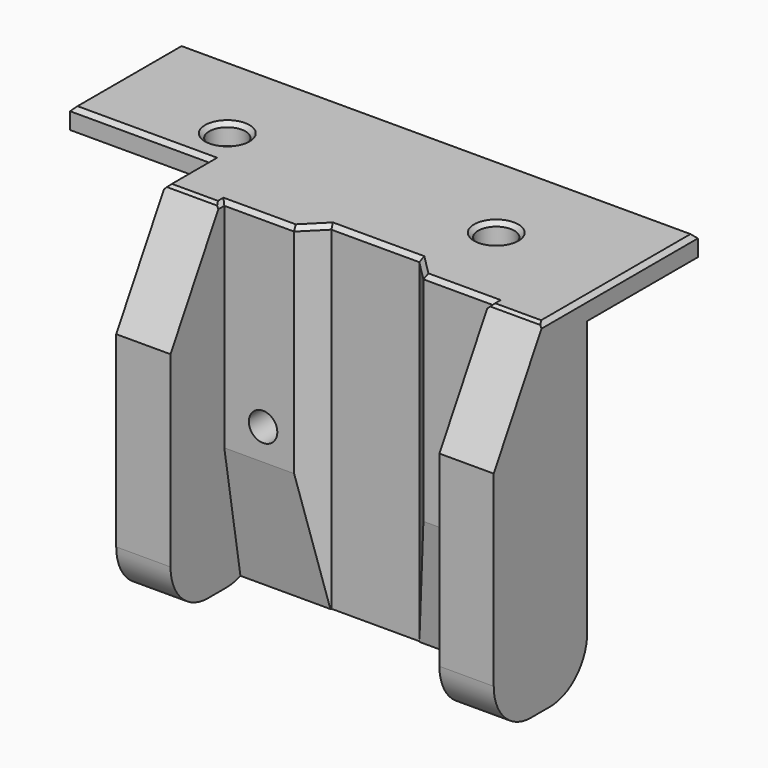
from build123d import *

# Parameters (mm, degrees)
F0_W           = 13.375
F0_H           = 2
F1_DEPTH       = 25
F2_R           = 1.75
F3_DEPTH       = 2
F4_W           = 11.3
F4_H           = 33
F5_DEPTH       = 25
F5_DEPTH_BACK  = 11.5
F6_W           = 26
F6_H           = 6.5
F7_DEPTH       = 33
F9_DEPTH       = 33
F11_DEPTH      = 19.75
F11_DEPTH_BACK = 6.25
F12_R          = 1.375
F13_DEPTH      = 4.8
F14_W          = 5.5
F14_H          = 5.5
F15_DEPTH      = 1.5
F16_T1_DEPTH   = 27.75
F16_T3_DEPTH   = 27.75
F16_T5_DEPTH   = 59
F17_T1_DEPTH   = 59.021567647
F17_T3_DEPTH   = 59.021567647
F18_T1_DEPTH   = 6.4746360003
F18_T3_DEPTH   = 20.7323463904
F18_T5_DEPTH   = 52.0573463904
F18_T7_DEPTH   = 15.4323463904
F18_T9_DEPTH   = 14.5286731952
F18_T11_DEPTH  = 6.3286731952
F18_T13_DEPTH  = 6.4746360003
F18_T15_DEPTH  = 1.5286731952
F18_T17_DEPTH  = 7.7786731952
F18_T19_DEPTH  = 7.7786731952
F18_T24_DEPTH  = 4.8857735151
F18_T29_DEPTH  = 10.5573463904
F18_T35_DEPTH  = 4.8857735151
F18_T45_DEPTH  = 14.5286731952
F18_T49_DEPTH  = 7.3573463904
F18_T56_DEPTH  = 8.8073463904
F18_T60_DEPTH  = 2.5573463904
F18_T67_DEPTH  = 4.8857735151
F18_T71_DEPTH  = 10.5573463904
F18_T78_DEPTH  = 10.5573463904
F18_T82_DEPTH  = 4.8857735151
F18_T89_DEPTH  = 2.5573463904
F18_T93_DEPTH  = 8.8073463904


# Not quite as in the source:
# - a fillet or chamfer that OpenCascade refuses, or shapes differently, is made with other operations: its cross-section is extruded or revolved along the edge and cut away or added


with BuildPart() as f1:
    # F0 (on Right) → F1 (new body, symmetric)
    with BuildSketch(Plane.YZ):
        with Locations((6.6875, 1)):
            Rectangle(F0_W, F0_H)
    extrude(amount=F1_DEPTH, both=True)

    # F2 (on face) → F3 (cut, through all)
    with BuildSketch(Plane.XY.offset(2)):
        with Locations((-13, 4)):
            Circle(F2_R)
        with Locations((13, 4)):
            Circle(F2_R)
    extrude(amount=-F3_DEPTH, mode=Mode.SUBTRACT)

    # F4 (on Right) → F5 (join, two sides)
    with BuildSketch(Plane.YZ) as f5_sk:
        with Locations((-5.65, -14.5)):
            Rectangle(F4_W, F4_H)
    extrude(amount=F5_DEPTH)
    extrude(f5_sk.sketch, amount=-F5_DEPTH_BACK)

    # F6 (on face) → F7 (cut, through all)
    with BuildSketch(Plane(origin=(0, 0, -31), x_dir=(1, 0, 0), z_dir=(0, 0, -1))):
        with Locations((6.75, 8.05)):
            Rectangle(F6_W, F6_H)
    extrude(amount=-F7_DEPTH, mode=Mode.SUBTRACT)

    # F8 (on face) → F9 (cut, through all)
    with BuildSketch(Plane(origin=(0, 0, -31), x_dir=(1, 0, 0), z_dir=(0, 0, -1))):
        Polygon((13, 4.8), (0.5, 4.8), (2.5, 2.8), (11, 2.8), align=None)
    extrude(amount=-F9_DEPTH, mode=Mode.SUBTRACT)

    # F10 (on Right) → F11 (cut, two sides)
    with BuildSketch(Plane.YZ) as f11_sk:
        Polygon((-4.8, -31), (-2.8, -31), (-4.8, -19), align=None)
    extrude(amount=F11_DEPTH, mode=Mode.SUBTRACT)
    extrude(f11_sk.sketch, amount=-F11_DEPTH_BACK, mode=Mode.SUBTRACT)

    # F12 (on face) → F13 (cut, through all)
    with BuildSketch(Plane.XZ.offset(4.8)):
        with Locations((-2.5, -16)):
            Circle(F12_R)
        with Locations((16, -16)):
            Circle(F12_R)
    extrude(amount=-F13_DEPTH, mode=Mode.SUBTRACT)

    # F14 (on face) → F15 (cut)
    with BuildSketch(Plane(origin=(0, 0, 0), x_dir=(-1, 0, 0), z_dir=(0, 1, 0))):
        with Locations((-16, -16)):
            Rectangle(F14_W, F14_H)
        with Locations((2.5, -16)):
            Rectangle(F14_W, F14_H)
    extrude(amount=-F15_DEPTH, mode=Mode.SUBTRACT)

    # F16: fillet of radius 4.5 on 3 edges, made by hand

    # F16_s2 → F16_t1 (cut)
    with BuildSketch(Plane.YZ.offset(-22.75)):
        with BuildLine():
            ThreePointArc((-11.3, -26.5), (-9.9819805153, -29.6819805153), (-6.8, -31))
            Line((-6.8, -31), (-11.3, -31))
            Line((-11.3, -31), (-11.3, -26.5))
        make_face()
    extrude(amount=F16_T1_DEPTH, mode=Mode.SUBTRACT)

    # F16_s4 → F16_t3 (cut)
    with BuildSketch(Plane.YZ.offset(8.5)):
        with BuildLine():
            ThreePointArc((-11.3, -26.5), (-9.9819805153, -29.6819805153), (-6.8, -31))
            Line((-6.8, -31), (-11.3, -31))
            Line((-11.3, -31), (-11.3, -26.5))
        make_face()
    extrude(amount=F16_T3_DEPTH, mode=Mode.SUBTRACT)

    # F16_s6 → F16_t5 (cut)
    with BuildSketch(Plane.YZ.offset(-22.75)):
        with BuildLine():
            ThreePointArc((0, -26.5), (-1.3180194847, -29.6819805153), (-4.5, -31))
            Line((-4.5, -31), (0, -31))
            Line((0, -31), (0, -26.5))
        make_face()
    extrude(amount=F16_T5_DEPTH, mode=Mode.SUBTRACT)

    # F17: chamfer of 6 x 10.3923048454 on 2 edges, made by hand

    # F17_s2 → F17_t1 (cut)
    with BuildSketch(Plane.YZ.offset(-38.3857838235)):
        Polygon((-5.3, 2), (-11.3, -8.3923048454), (-11.3, 2), align=None)
    extrude(amount=F17_T1_DEPTH, mode=Mode.SUBTRACT)

    # F17_s4 → F17_t3 (cut)
    with BuildSketch(Plane.YZ.offset(-7.1357838235)):
        Polygon((-5.3, 2), (-11.3, -8.3923048454), (-11.3, 2), align=None)
    extrude(amount=F17_T3_DEPTH, mode=Mode.SUBTRACT)

    # F18: chamfer of 0.4 on 16 edges, made by hand

    # F18_s2 → F18_t1 (cut)
    with BuildSketch(Plane.YZ.offset(19.1376819998)):
        Polygon((-5.4154700538, 1.8), (-5.0690598923, 2), (-5.3, 2), align=None)
    extrude(amount=F18_T1_DEPTH, mode=Mode.SUBTRACT)

    # F18_s4 → F18_t3 (cut)
    with BuildSketch(Plane.XZ.offset(-14.4036731952)):
        Polygon((25, 1.6), (24.6, 2), (25, 2), align=None)
    extrude(amount=F18_T3_DEPTH, mode=Mode.SUBTRACT)

    # F18_s6 → F18_t5 (cut)
    with BuildSketch(Plane.YZ.offset(-26.0286731952)):
        Polygon((13.375, 1.6), (12.975, 2), (13.375, 2), align=None)
    extrude(amount=F18_T5_DEPTH, mode=Mode.SUBTRACT)

    # F18_s8 → F18_t7 (cut)
    with BuildSketch(Plane.XZ.offset(-14.4036731952)):
        Polygon((-25, 1.6), (-24.6, 2), (-25, 2), align=None)
    extrude(amount=F18_T7_DEPTH, mode=Mode.SUBTRACT)

    # F18_s10 → F18_t9 (cut)
    with BuildSketch(Plane.YZ.offset(-26.0286731952)):
        Polygon((0, 1.6), (0.4, 2), (0, 2), align=None)
    extrude(amount=F18_T9_DEPTH, mode=Mode.SUBTRACT)

    # F18_s12 → F18_t11 (cut)
    with BuildSketch(Plane.XZ):
        Polygon((-11.5, 1.6), (-11.1, 2), (-11.5, 2), align=None)
    extrude(amount=F18_T11_DEPTH, mode=Mode.SUBTRACT)

    # F18_s14 → F18_t13 (cut)
    with BuildSketch(Plane.YZ.offset(-12.1123180002)):
        Polygon((-5.4154700538, 1.8), (-5.0690598923, 2), (-5.3, 2), align=None)
    extrude(amount=F18_T13_DEPTH, mode=Mode.SUBTRACT)

    # F18_s16 → F18_t15 (cut)
    with BuildSketch(Plane.XZ.offset(4.8)):
        Polygon((-6.25, 1.6), (-6.65, 2), (-6.25, 2), align=None)
        Polygon((19.75, 1.6), (20.15, 2), (19.75, 2), align=None)
    extrude(amount=F18_T15_DEPTH, mode=Mode.SUBTRACT)

    # F18_s18 → F18_t17 (cut)
    with BuildSketch(Plane.YZ.offset(-6.25)):
        Polygon((-4.8, 1.6), (-4.4, 2), (-4.8, 2), align=None)
    extrude(amount=F18_T17_DEPTH, mode=Mode.SUBTRACT)

    # F18_s20 → F18_t19 (cut)
    with BuildSketch(Plane.YZ.offset(11.9713268048)):
        Polygon((-4.8, 1.6), (-4.4, 2), (-4.8, 2), align=None)
    extrude(amount=F18_T19_DEPTH, mode=Mode.SUBTRACT)


with BuildPart() as f18_tool22:
    # F18_s23 → F18_t24 (new body)
    with BuildSketch(Plane(origin=(-2.8773817919, -2.8773817919, 0), x_dir=(0, 0, 1), z_dir=(0.7071067812, 0.7071067812, 0))):
        Polygon((1.6, 3.7476659403), (2, 3.3476659403), (2, 3.7476659403), align=None)
    extrude(amount=F18_T24_DEPTH)

    split(bisect_by=Plane.XZ.offset(2.8), keep=Keep.TOP)


with BuildPart() as f1_1:
    add(f1.part)

    # F18_t21: cut F18_tool22
    add(f18_tool22.part, mode=Mode.SUBTRACT)


with BuildPart() as f18_tool27:
    # F18_s28 → F18_t29 (new body)
    with BuildSketch(Plane.YZ.offset(1.4713268048)):
        Polygon((-2.8, 1.6), (-2.4, 2), (-2.8, 2), align=None)
    extrude(amount=F18_T29_DEPTH)

    split(bisect_by=Plane(origin=(2.65, -2.65, 0), x_dir=(0, 0, 1), z_dir=(0.7071067812, -0.7071067812, 0)), keep=Keep.TOP)

    split(bisect_by=Plane(origin=(4.1, 4.1, 0), x_dir=(0, 0, 1), z_dir=(-0.7071067812, -0.7071067812, 0)), keep=Keep.TOP)


with BuildPart() as f1_2:
    add(f1_1.part)

    # F18_t26: cut F18_tool27
    add(f18_tool27.part, mode=Mode.SUBTRACT)


with BuildPart() as f18_tool33:
    # F18_s34 → F18_t35 (new body)
    with BuildSketch(Plane(origin=(6.1726182081, -6.1726182081, 0), x_dir=(0, 0, 1), z_dir=(0.7071067812, -0.7071067812, 0))):
        Polygon((1.6, -5.7982756057), (2, -6.1982756057), (2, -5.7982756057), align=None)
    extrude(amount=F18_T35_DEPTH)

    split(bisect_by=Plane.XZ.offset(2.8), keep=Keep.TOP)


with BuildPart() as f1_3:
    add(f1_2.part)

    # F18_t32: cut F18_tool33
    add(f18_tool33.part, mode=Mode.SUBTRACT)

    # F18_s37 → F18_t38 (revolve, cut)
    with BuildSketch(Plane.XZ.offset(-4)):
        Polygon((-11.25, 1.6), (-10.85, 2), (-11.25, 2), align=None)
    revolve(axis=Axis((-13, 4, 2), (0, 0, 1)), mode=Mode.SUBTRACT)

    # F18_s39 → F18_t40 (revolve, cut)
    with BuildSketch(Plane.XZ.offset(-4)):
        Polygon((14.75, 1.6), (15.15, 2), (14.75, 2), align=None)
    revolve(axis=Axis((13, 4, 2), (0, 0, 1)), mode=Mode.SUBTRACT)


with BuildPart() as f18_tool43:
    # F18_s44 → F18_t45 (new body)
    with BuildSketch(Plane.YZ.offset(-10.4713268048)):
        Polygon((0, 1.6), (0.4, 2), (0, 2), align=None)
    extrude(amount=-F18_T45_DEPTH)

    split(bisect_by=Plane.YZ.offset(-11.5), keep=Keep.TOP)


with BuildPart() as f18_tool47:
    # F18_s48 → F18_t49 (new body)
    with BuildSketch(Plane.XZ.offset(-1.0286731952)):
        Polygon((-11.5, 1.6), (-11.1, 2), (-11.5, 2), align=None)
    extrude(amount=F18_T49_DEPTH)

    split(bisect_by=Plane.XZ, keep=Keep.BOTTOM)


with BuildPart() as f18_tool43_1:
    add(f18_tool43.part)

    # F18_t51: intersect F18_tool47
    add(f18_tool47.part, mode=Mode.INTERSECT)


with BuildPart() as f1_4:
    add(f1_3.part)

    # F18_t41: cut F18_tool43
    add(f18_tool43_1.part, mode=Mode.SUBTRACT)


with BuildPart() as f18_tool54:
    # F18_s55 → F18_t56 (new body)
    with BuildSketch(Plane.YZ.offset(-7.2786731952)):
        Polygon((-4.8, 1.6), (-4.4, 2), (-4.8, 2), align=None)
    extrude(amount=F18_T56_DEPTH)

    split(bisect_by=Plane.YZ.offset(-6.25), keep=Keep.BOTTOM)


with BuildPart() as f18_tool58:
    # F18_s59 → F18_t60 (new body)
    with BuildSketch(Plane.XZ.offset(6.3286731952)):
        Polygon((-6.25, 1.6), (-6.65, 2), (-6.25, 2), align=None)
    extrude(amount=-F18_T60_DEPTH)

    split(bisect_by=Plane.XZ.offset(4.8), keep=Keep.BOTTOM)


with BuildPart() as f18_tool54_1:
    add(f18_tool54.part)

    # F18_t62: intersect F18_tool58
    add(f18_tool58.part, mode=Mode.INTERSECT)


with BuildPart() as f1_5:
    add(f1_4.part)

    # F18_t52: cut F18_tool54
    add(f18_tool54_1.part, mode=Mode.SUBTRACT)


with BuildPart() as f18_tool65:
    # F18_s66 → F18_t67 (new body)
    with BuildSketch(Plane(origin=(-2.8773817919, -2.8773817919, 0), x_dir=(0, 0, 1), z_dir=(0.7071067812, 0.7071067812, 0))):
        Polygon((1.6, 3.7476659403), (2, 3.3476659403), (2, 3.7476659403), align=None)
    extrude(amount=F18_T67_DEPTH)

    split(bisect_by=Plane.XZ.offset(2.8), keep=Keep.BOTTOM)


with BuildPart() as f18_tool69:
    # F18_s70 → F18_t71 (new body)
    with BuildSketch(Plane.YZ.offset(1.4713268048)):
        Polygon((-2.8, 1.6), (-2.4, 2), (-2.8, 2), align=None)
    extrude(amount=F18_T71_DEPTH)

    split(bisect_by=Plane(origin=(2.65, -2.65, 0), x_dir=(0, 0, 1), z_dir=(-0.7071067812, 0.7071067812, 0)), keep=Keep.TOP)


with BuildPart() as f18_tool65_1:
    add(f18_tool65.part)

    # F18_t73: intersect F18_tool69
    add(f18_tool69.part, mode=Mode.INTERSECT)


with BuildPart() as f1_6:
    add(f1_5.part)

    # F18_t63: cut F18_tool65
    add(f18_tool65_1.part, mode=Mode.SUBTRACT)


with BuildPart() as f18_tool76:
    # F18_s77 → F18_t78 (new body)
    with BuildSketch(Plane.YZ.offset(1.4713268048)):
        Polygon((-2.8, 1.6), (-2.4, 2), (-2.8, 2), align=None)
    extrude(amount=F18_T78_DEPTH)

    split(bisect_by=Plane(origin=(4.1, 4.1, 0), x_dir=(0, 0, 1), z_dir=(0.7071067812, 0.7071067812, 0)), keep=Keep.TOP)


with BuildPart() as f18_tool80:
    # F18_s81 → F18_t82 (new body)
    with BuildSketch(Plane(origin=(6.1726182081, -6.1726182081, 0), x_dir=(0, 0, 1), z_dir=(0.7071067812, -0.7071067812, 0))):
        Polygon((1.6, -5.7982756057), (2, -6.1982756057), (2, -5.7982756057), align=None)
    extrude(amount=F18_T82_DEPTH)

    split(bisect_by=Plane.XZ.offset(2.8), keep=Keep.BOTTOM)


with BuildPart() as f18_tool76_1:
    add(f18_tool76.part)

    # F18_t84: intersect F18_tool80
    add(f18_tool80.part, mode=Mode.INTERSECT)


with BuildPart() as f1_7:
    add(f1_6.part)

    # F18_t74: cut F18_tool76
    add(f18_tool76_1.part, mode=Mode.SUBTRACT)


with BuildPart() as f18_tool87:
    # F18_s88 → F18_t89 (new body)
    with BuildSketch(Plane.XZ.offset(3.7713268048)):
        Polygon((19.75, 1.6), (20.15, 2), (19.75, 2), align=None)
    extrude(amount=F18_T89_DEPTH)

    split(bisect_by=Plane.XZ.offset(4.8), keep=Keep.BOTTOM)


with BuildPart() as f18_tool91:
    # F18_s92 → F18_t93 (new body)
    with BuildSketch(Plane.YZ.offset(11.9713268048)):
        Polygon((-4.8, 1.6), (-4.4, 2), (-4.8, 2), align=None)
    extrude(amount=F18_T93_DEPTH)

    split(bisect_by=Plane.YZ.offset(19.75), keep=Keep.TOP)


with BuildPart() as f18_tool87_1:
    add(f18_tool87.part)

    # F18_t95: intersect F18_tool91
    add(f18_tool91.part, mode=Mode.INTERSECT)


with BuildPart() as f1_8:
    add(f1_7.part)

    # F18_t85: cut F18_tool87
    add(f18_tool87_1.part, mode=Mode.SUBTRACT)


solid = f1_8.part
